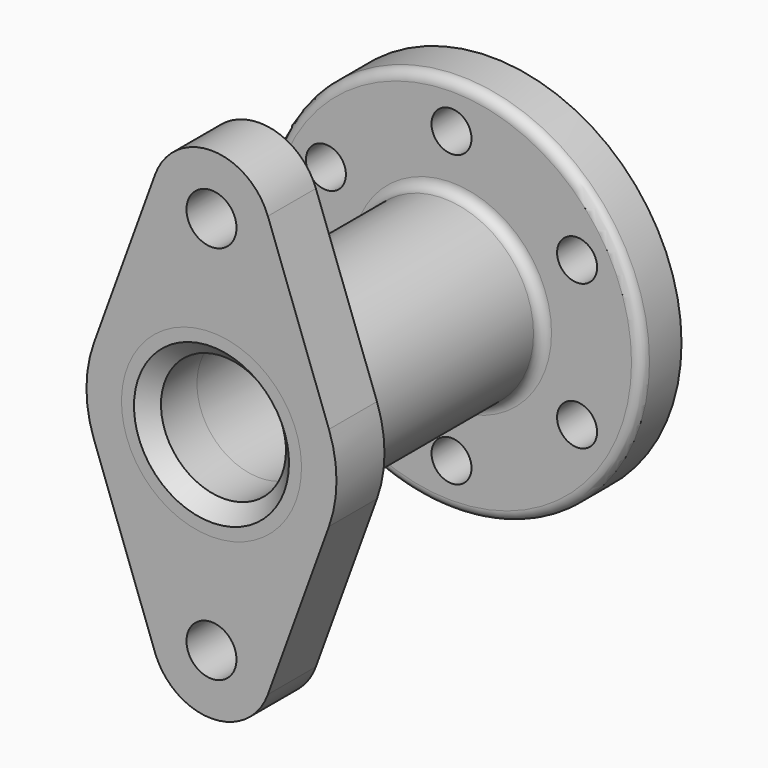
from build123d import *

# Parameters (mm, degrees)
F0_R      = 965.2
F1_DEPTH  = 254
F2_D      = 203.2
F3_R      = 457.2
F3_R_2    = 317.5
F4_DEPTH  = 1219.2
F5_R      = 50.8
F3_R_3    = 254
F6_DEPTH  = 254.001
F7_DEPTH  = 584.2
F10_DEPTH = 304.8
F11_DEPTH = 304.8
F12_SIZE2 = 76.2
F12_SIZE  = 76.2


# Not quite as in the source:
# - a feature names something its author has since deleted; it is built from what else it names


with BuildPart() as f1:
    # F0 (on Front) → F1 (new body)
    with BuildSketch(Plane.XZ):
        Circle(F0_R)
        with BuildLine():
            ThreePointArc((682.5252094596, 277.017866666), (722.9549188186, 141.1231566967), (736.6, 0))
            ThreePointArc((736.6, 0), (722.9549188186, -141.1231566967), (682.5252094596, -277.017866666))
            ThreePointArc((682.5252094596, -277.017866666), (724.0973360995, -314.4943643214), (739.5143124276, -368.3))
            ThreePointArc((739.5143124276, -368.3), (685.6481824631, -457.9885592004), (581.1671145647, -452.5752367823))
            ThreePointArc((581.1671145647, -452.5752367823), (368.3, -637.9143124276), (101.3580948948, -729.5931034483))
            ThreePointArc((101.3580948949, -729.5931034483), (101.5395057141, -733.0944644715), (101.6, -736.6))
            ThreePointArc((101.6, -736.6), (-3.5055355285, -838.1395057141), (-101.3580948949, -729.5931034483))
            ThreePointArc((-101.3580948948, -729.5931034483), (-368.3, -637.9143124276), (-581.1671145647, -452.5752367823))
            ThreePointArc((-581.1671145647, -452.5752367823), (-725.9024934521, -419.1), (-682.5252094596, -277.017866666))
            ThreePointArc((-682.5252094596, -277.017866666), (-736.6, 0), (-682.5252094596, 277.017866666))
            ThreePointArc((-682.5252094596, 277.017866666), (-725.9024934521, 419.1), (-581.1671145647, 452.5752367823))
            ThreePointArc((-581.1671145647, 452.5752367823), (-368.3, 637.9143124276), (-101.3580948948, 729.5931034483))
            ThreePointArc((-101.3580948949, 729.5931034483), (-3.5055355285, 838.1395057141), (101.6, 736.6))
            ThreePointArc((101.6, 736.6), (101.5395057141, 733.0944644715), (101.3580948949, 729.5931034483))
            ThreePointArc((101.3580948948, 729.5931034483), (368.3, 637.9143124276), (581.1671145647, 452.5752367823))
            ThreePointArc((581.1671145647, 452.5752367823), (685.6481824631, 457.9885592004), (739.5143124276, 368.3))
            ThreePointArc((739.5143124276, 368.3), (724.0973360995, 314.4943643214), (682.5252094596, 277.017866666))
        make_face(mode=Mode.SUBTRACT)
        with BuildLine():
            ThreePointArc((682.5252094596, -277.017866666), (722.9549188186, -141.1231566967), (736.6, 0))
            ThreePointArc((736.6, 0), (722.9549188186, 141.1231566967), (682.5252094596, 277.017866666))
            ThreePointArc((682.5252094596, 277.017866666), (549.9261314031, 317.5), (581.1671145647, 452.5752367823))
            ThreePointArc((581.1671145647, 452.5752367823), (368.3, 637.9143124276), (101.3580948948, 729.5931034483))
            ThreePointArc((101.3580948949, 729.5931034483), (0, 635), (-101.3580948949, 729.5931034483))
            ThreePointArc((-101.3580948948, 729.5931034483), (-368.3, 637.9143124276), (-581.1671145647, 452.5752367823))
            ThreePointArc((-581.1671145647, 452.5752367823), (-548.2257532273, 416.0338700355), (-536.3143124276, 368.3))
            ThreePointArc((-536.3143124276, 368.3), (-584.108676749, 282.1169763282), (-682.5252094596, 277.017866666))
            ThreePointArc((-682.5252094596, 277.017866666), (-736.6, 0), (-682.5252094596, -277.017866666))
            ThreePointArc((-682.5252094596, -277.017866666), (-584.108676749, -282.1169763282), (-536.3143124276, -368.3))
            ThreePointArc((-536.3143124276, -368.3), (-548.2257532273, -416.0338700355), (-581.1671145647, -452.5752367823))
            ThreePointArc((-581.1671145647, -452.5752367823), (-368.3, -637.9143124276), (-101.3580948948, -729.5931034483))
            ThreePointArc((-101.3580948949, -729.5931034483), (0, -635), (101.3580948949, -729.5931034483))
            ThreePointArc((101.3580948948, -729.5931034483), (368.3, -637.9143124276), (581.1671145647, -452.5752367823))
            ThreePointArc((581.1671145647, -452.5752367823), (549.9261314031, -317.5), (682.5252094596, -277.017866666))
        make_face()
        with BuildLine():
            ThreePointArc((-682.5252094596, 277.017866666), (-637.9143124276, 368.3), (-581.1671145647, 452.5752367823))
            ThreePointArc((-581.1671145647, 452.5752367823), (-725.9024934521, 419.1), (-682.5252094596, 277.017866666))
        make_face()
        with BuildLine():
            ThreePointArc((-101.3580948948, 729.5931034483), (0, 736.6), (101.3580948948, 729.5931034483))
            ThreePointArc((101.3580948949, 729.5931034483), (101.5395057141, 733.0944644715), (101.6, 736.6))
            ThreePointArc((101.6, 736.6), (-3.5055355285, 838.1395057141), (-101.3580948949, 729.5931034483))
        make_face()
        with BuildLine():
            ThreePointArc((-682.5252094596, -277.017866666), (-725.9024934521, -419.1), (-581.1671145647, -452.5752367823))
            ThreePointArc((-581.1671145647, -452.5752367823), (-637.9143124276, -368.3), (-682.5252094596, -277.017866666))
        make_face()
        with BuildLine():
            ThreePointArc((101.6, -736.6), (101.5395057141, -733.0944644715), (101.3580948949, -729.5931034483))
            ThreePointArc((101.3580948948, -729.5931034483), (0, -736.6), (-101.3580948948, -729.5931034483))
            ThreePointArc((-101.3580948949, -729.5931034483), (-3.5055355285, -838.1395057141), (101.6, -736.6))
        make_face()
        with BuildLine():
            ThreePointArc((739.5143124276, -368.3), (724.0973360995, -314.4943643214), (682.5252094596, -277.017866666))
            ThreePointArc((682.5252094596, -277.017866666), (637.9143124276, -368.3), (581.1671145647, -452.5752367823))
            ThreePointArc((581.1671145647, -452.5752367823), (685.6481824631, -457.9885592004), (739.5143124276, -368.3))
        make_face()
        with BuildLine():
            ThreePointArc((581.1671145647, 452.5752367823), (637.9143124276, 368.3), (682.5252094596, 277.017866666))
            ThreePointArc((682.5252094596, 277.017866666), (724.0973360995, 314.4943643214), (739.5143124276, 368.3))
            ThreePointArc((739.5143124276, 368.3), (685.6481824631, 457.9885592004), (581.1671145647, 452.5752367823))
        make_face()
        with BuildLine():
            ThreePointArc((-536.3143124276, 368.3), (-548.2257532273, 416.0338700355), (-581.1671145647, 452.5752367823))
            ThreePointArc((-581.1671145647, 452.5752367823), (-637.9143124276, 368.3), (-682.5252094596, 277.017866666))
            ThreePointArc((-682.5252094596, 277.017866666), (-584.108676749, 282.1169763282), (-536.3143124276, 368.3))
        make_face()
        with BuildLine():
            ThreePointArc((-101.3580948949, 729.5931034483), (0, 635), (101.3580948949, 729.5931034483))
            ThreePointArc((101.3580948948, 729.5931034483), (0, 736.6), (-101.3580948948, 729.5931034483))
        make_face()
        with BuildLine():
            ThreePointArc((-682.5252094596, -277.017866666), (-637.9143124276, -368.3), (-581.1671145647, -452.5752367823))
            ThreePointArc((-581.1671145647, -452.5752367823), (-548.2257532273, -416.0338700355), (-536.3143124276, -368.3))
            ThreePointArc((-536.3143124276, -368.3), (-584.108676749, -282.1169763282), (-682.5252094596, -277.017866666))
        make_face()
        with BuildLine():
            ThreePointArc((-101.3580948948, -729.5931034483), (0, -736.6), (101.3580948948, -729.5931034483))
            ThreePointArc((101.3580948949, -729.5931034483), (0, -635), (-101.3580948949, -729.5931034483))
        make_face()
        with BuildLine():
            ThreePointArc((581.1671145647, -452.5752367823), (637.9143124276, -368.3), (682.5252094596, -277.017866666))
            ThreePointArc((682.5252094596, -277.017866666), (549.9261314031, -317.5), (581.1671145647, -452.5752367823))
        make_face()
        with BuildLine():
            ThreePointArc((581.1671145647, 452.5752367823), (549.9261314031, 317.5), (682.5252094596, 277.017866666))
            ThreePointArc((682.5252094596, 277.017866666), (637.9143124276, 368.3), (581.1671145647, 452.5752367823))
        make_face()
    extrude(amount=F1_DEPTH)

    # F2 (through all)
    with Locations(Plane(origin=(0, 0, 0), x_dir=(1, 0, 0), z_dir=(0, 1, 0))):
        with Locations((0, -736.6), (-637.9143124276, -368.3), (-637.9143124276, 368.3), (0, 736.6), (637.9143124276, 368.3), (637.9143124276, -368.3)):
            Hole(F2_D / 2)

    # F3 (on face) → F4 (join)
    with BuildSketch(Plane.XZ.offset(254)):
        Circle(F3_R)
        Circle(F3_R_2, mode=Mode.SUBTRACT)
    extrude(amount=F4_DEPTH)

    # F5
    f5_edges = [f1.edges().sort_by_distance(p)[0] for p in [
        (-965.2, -254, 0),
        (-457.2, -254, 0),
    ]]
    fillet(f5_edges, radius=F5_R)

    # F3 (on face) → F6 (cut, through all)
    with BuildSketch(Plane.XZ.offset(254)):
        Circle(F3_R_3)
    extrude(amount=-F6_DEPTH, mode=Mode.SUBTRACT)

    # F3 (on face) → F7 (join)
    with BuildSketch(Plane.XZ.offset(254)):
        Circle(F3_R_2)
        Circle(F3_R_3, mode=Mode.SUBTRACT)
    extrude(amount=F7_DEPTH)

    # F9 (on face) → F10 (join)
    with BuildSketch(Plane.XZ.offset(1473.2)):
        with BuildLine():
            ThreePointArc((0, 660.4), (215.5261469057, 749.6738530943), (304.8, 965.2))
            ThreePointArc((304.8, 965.2), (300.1670055935, 1018.1415597902), (286.40886645, 1069.4736842105))
            ThreePointArc((286.40886645, 1069.4736842105), (0, 1270), (-286.40886645, 1069.4736842105))
            ThreePointArc((-286.40886645, 1069.4736842105), (-249.6854610779, 790.3852107906), (0, 660.4))
        make_face()
        with BuildLine():
            ThreePointArc((127, 965.2), (89.8025612107, 875.3974387893), (0, 838.2))
            ThreePointArc((0, 838.2), (-89.8025612107, 1055.0025612107), (127, 965.2))
        make_face(mode=Mode.SUBTRACT)
        with BuildLine():
            ThreePointArc((286.40886645, 1069.4736842105), (300.1670055935, 1018.1415597902), (304.8, 965.2))
            ThreePointArc((304.8, 965.2), (215.5261469057, 749.6738530943), (0, 660.4))
            Line((0, 660.4), (0, 635))
            ThreePointArc((0, 635), (364.1974814541, 520.1780411576), (596.6851417238, 217.2368330788))
            Line((596.6851417238, 217.2368330788), (286.40886645, 1069.4736842105))
        make_face()
        with BuildLine():
            Line((0, 635), (0, 660.4))
            ThreePointArc((0, 660.4), (-249.6854610779, 790.3852107906), (-286.40886645, 1069.4736842105))
            Line((-286.40886645, 1069.4736842105), (-596.6851384375, 217.2368421053))
            ThreePointArc((-596.6851384375, 217.2368421053), (-364.1974775195, 520.1780439123), (0, 635))
        make_face()
        with BuildLine():
            ThreePointArc((635, 0), (625.3479291541, 110.2949114996), (596.6851417238, 217.2368330788))
            ThreePointArc((596.6851417238, 217.2368330788), (364.1974814541, 520.1780411576), (0, 635))
            Line((0, 635), (0, 457.2))
            Line((0, 457.2), (0, 330.2))
            ThreePointArc((0, 330.2), (233.4866591478, 233.4866591478), (330.2, 0))
            ThreePointArc((330.2, 0), (233.4866591478, -233.4866591478), (0, -330.2))
            Line((0, -330.2), (0, -635))
            ThreePointArc((0, -635), (364.1974775195, -520.1780439123), (596.6851384375, -217.2368421053))
            ThreePointArc((596.6851384375, -217.2368421053), (625.3479283198, -110.2949162297), (635, 0))
        make_face()
        with BuildLine():
            Line((0, 457.2), (0, 635))
            ThreePointArc((0, 635), (-364.1974775195, 520.1780439123), (-596.6851384375, 217.2368421053))
            ThreePointArc((-596.6851384375, 217.2368421053), (-635, 4.0958e-06), (-596.6851412398, -217.236834408))
            ThreePointArc((-596.6851412398, -217.236834408), (-364.1974808747, -520.1780415632), (0, -635))
            Line((0, -635), (0, -330.2))
            ThreePointArc((0, -330.2), (-233.4866591478, -233.4866591478), (-330.2, 0))
            Line((-330.2, 0), (-457.2, 0))
            ThreePointArc((-457.2, 0), (-323.2892203585, 323.2892203585), (0, 457.2))
        make_face()
        with BuildLine():
            Line((0, 330.2), (0, 457.2))
            ThreePointArc((0, 457.2), (-323.2892203585, 323.2892203585), (-457.2, 0))
            Line((-457.2, 0), (-330.2, 0))
            ThreePointArc((-330.2, 0), (-233.4866591478, 233.4866591478), (0, 330.2))
        make_face()
        with BuildLine():
            ThreePointArc((0, -635), (-364.1974808747, -520.1780415632), (-596.6851412398, -217.236834408))
            Line((-596.6851412398, -217.236834408), (-286.40886645, -1069.4736842105))
            ThreePointArc((-286.40886645, -1069.4736842105), (-249.6854610779, -790.3852107906), (0, -660.4))
            Line((0, -660.4), (0, -635))
        make_face()
        with BuildLine():
            Line((286.4088669044, -1069.4736829624), (596.6851384375, -217.2368421053))
            ThreePointArc((596.6851384375, -217.2368421053), (364.1974775195, -520.1780439123), (0, -635))
            Line((0, -635), (0, -660.4))
            ThreePointArc((0, -660.4), (215.5261469057, -749.6738530943), (304.8, -965.2))
            ThreePointArc((304.8, -965.2), (300.1670057089, -1018.1415591362), (286.4088669044, -1069.4736829624))
        make_face()
        with BuildLine():
            ThreePointArc((0, -660.4), (-249.6854610779, -790.3852107906), (-286.40886645, -1069.4736842105))
            ThreePointArc((-286.40886645, -1069.4736842105), (6.642e-07, -1270), (286.4088669044, -1069.4736829624))
            ThreePointArc((286.4088669044, -1069.4736829624), (300.1670057089, -1018.1415591362), (304.8, -965.2))
            ThreePointArc((304.8, -965.2), (215.5261469057, -749.6738530943), (0, -660.4))
        make_face()
        with BuildLine():
            ThreePointArc((127, -965.2), (-89.8025612107, -1055.0025612107), (0, -838.2))
            ThreePointArc((0, -838.2), (89.8025612107, -875.3974387893), (127, -965.2))
        make_face(mode=Mode.SUBTRACT)
    extrude(amount=F10_DEPTH)

    # F8 (on face) → F11 (join)
    with BuildSketch(Plane.XZ.offset(1473.2)):
        with BuildLine():
            Line((0, -457.2), (0, -317.5))
            ThreePointArc((0, -317.5), (-224.5064030267, -224.5064030267), (-317.5, 0))
            Line((-317.5, 0), (-457.2, 0))
            ThreePointArc((-457.2, 0), (-323.2892203585, -323.2892203585), (0, -457.2))
        make_face()
        with BuildLine():
            ThreePointArc((-317.5, 0), (-224.5064030267, 224.5064030267), (0, 317.5))
            Line((0, 317.5), (0, 457.2))
            ThreePointArc((0, 457.2), (-323.2892203585, 323.2892203585), (-457.2, 0))
            Line((-457.2, 0), (-317.5, 0))
        make_face()
        with BuildLine():
            Line((0, 457.2), (0, 317.5))
            ThreePointArc((0, 317.5), (224.5064030267, 224.5064030267), (317.5, 0))
            Line((317.5, 0), (457.2, 0))
            ThreePointArc((457.2, 0), (323.2892203585, 323.2892203585), (0, 457.2))
        make_face()
        with BuildLine():
            ThreePointArc((317.5, 0), (224.5064030267, -224.5064030267), (0, -317.5))
            Line((0, -317.5), (0, -457.2))
            ThreePointArc((0, -457.2), (323.2892203585, -323.2892203585), (457.2, 0))
            Line((457.2, 0), (317.5, 0))
        make_face()
    extrude(amount=F11_DEPTH)

    # F12
    f12_edges = [f1.edges().sort_by_distance(p)[0] for p in [
        (-317.5, -1778, 0),
    ]]
    chamfer(f12_edges, length=F12_SIZE, length2=F12_SIZE2)


solid = f1.part
